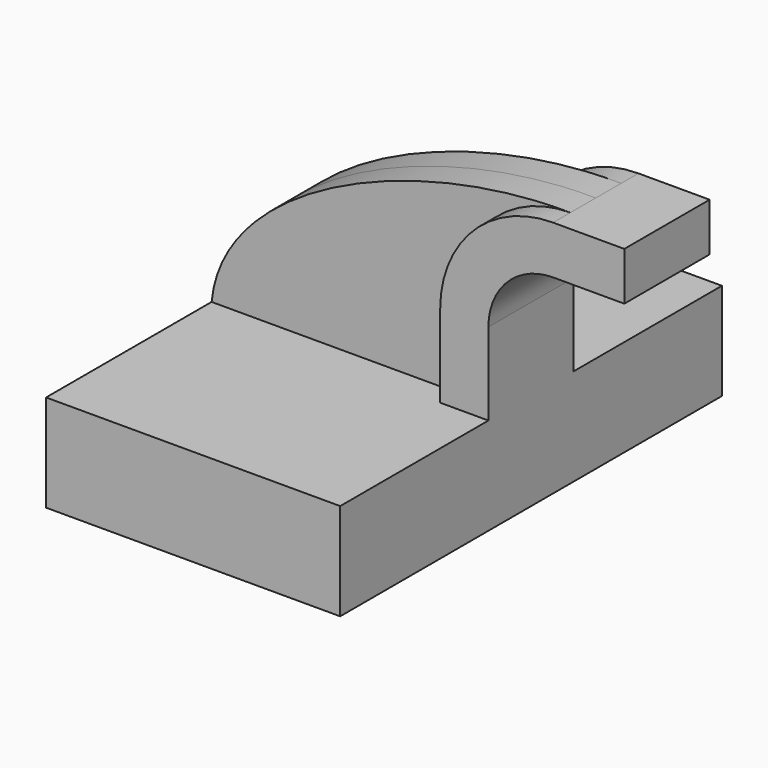
from build123d import *

# Parameters (mm, degrees)
F1_DEPTH = 40.56158
F2_DEPTH = 5.38948
F0_W     = 12.0462047143
F0_H     = 8.1998697145
F3_DEPTH = 9.06237


with BuildPart() as f1:
    # F0 (on Front) → F1 (new body, symmetric)
    with BuildSketch(Plane.XZ):
        Polygon((-14.8684419692, -13.1286175627), (-56.6685722546, -13.1286175627), (-56.6685722546, -29.630266222), (-6.6685722546, -29.630266222), (-6.6685722546, -13.1286175627), align=None)
    extrude(amount=F1_DEPTH, both=True)

    # F0 (on Front) → F2 (join, symmetric)
    with BuildSketch(Plane.XZ):
        with BuildLine():
            add(Edge.make_bspline(
                [(-56.6685722546, -13.1286175627), (-54.7797419131, 6.6462885588), (-22.0853742212, 20.4196609557), (4.3314277454, 20.0712521518)],
                knots=[0, 0, 0, 0, 69.4494877523, 69.4494877523, 69.4494877523, 69.4494877523], degree=3))
            Line((-56.6685722546, -13.1286175627), (-14.8684419692, -13.1286175627))
            Line((-14.8684419692, -13.1286175627), (-14.8684419692, 0.8713824373))
            ThreePointArc((-14.8684419692, 0.8713824373), (-9.2449303277, 14.4477405103), (4.3314277454, 20.0712521518))
        make_face()
    extrude(amount=F2_DEPTH, both=True)

    # F0 (on Front) → F3 (join, symmetric)
    with BuildSketch(Plane.XZ):
        with BuildLine():
            Line((-14.8684419692, 0.8713824373), (-14.8684419692, -13.1286175627))
            Line((-14.8684419692, -13.1286175627), (-6.6685722546, -13.1286175627))
            Line((-6.6685722546, -13.1286175627), (-6.6685722546, 0.8713824373))
            ThreePointArc((-6.6685722546, 0.8713824373), (-3.4467468477, 8.6495570304), (4.3314277454, 11.8713824373))
            Line((4.3314277454, 11.8713824373), (4.3880510932, 11.8713824373))
            Line((4.3880510932, 11.8713824373), (4.3880510932, 20.0712521518))
            Line((4.3880510932, 20.0712521518), (4.3314277454, 20.0712521518))
            ThreePointArc((4.3314277454, 20.0712521518), (-9.2449303277, 14.4477405103), (-14.8684419692, 0.8713824373))
        make_face()
        with Locations((10.4111534504, 15.9713172946)):
            Rectangle(F0_W, F0_H)
    extrude(amount=F3_DEPTH, both=True)


solid = f1.part
